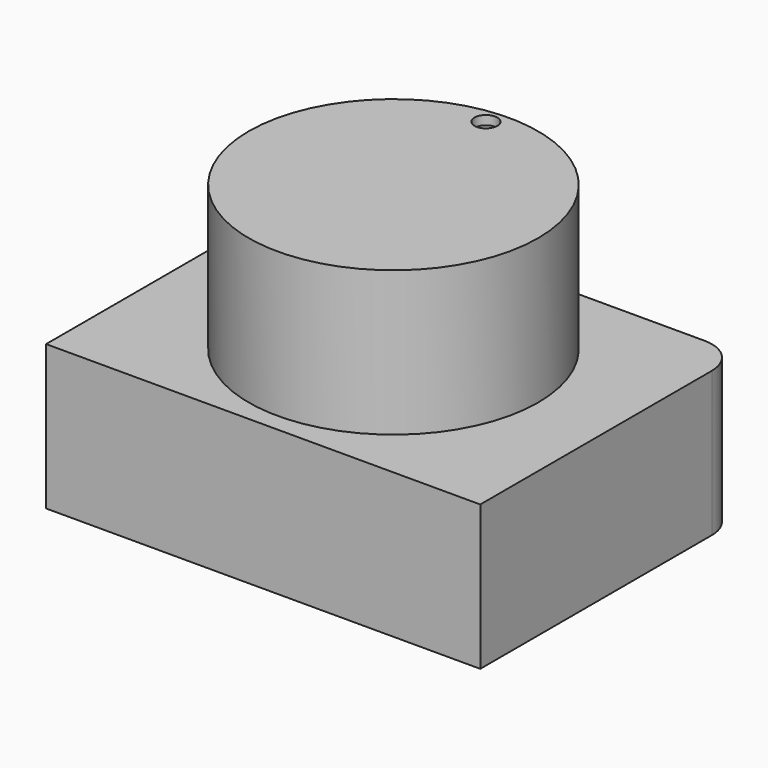
from build123d import *

# Parameters (mm, degrees)
F1_DEPTH = 25.4
F2_R     = 25.4
F3_DEPTH = 25.4
F6_DEPTH = 3.175
F7_R     = 1.9943268645
F8_DEPTH = 1.5875


# Not quite as in the source:
# - a feature of the source that left no trace in its solid (it failed there, or was rolled back) is left out


with BuildPart() as f1:
    # F0 (on Top) → F1 (new body)
    with BuildSketch(Plane.XY):
        with BuildLine():
            Line((-76.2, 0), (0, 0))
            Line((0, 0), (0, 50.8))
            ThreePointArc((0, 50.8), (-1.8598719395, 55.2901280605), (-6.35, 57.15))
            Line((-6.35, 57.15), (-69.85, 57.15))
            ThreePointArc((-69.85, 57.15), (-74.3401280605, 55.2901280605), (-76.2, 50.8))
            Line((-76.2, 50.8), (-76.2, 0))
        make_face()
    extrude(amount=F1_DEPTH)

    # F2 (on face) → F6 (cut)
    with BuildSketch(Plane.XY.offset(25.4)):
        with Locations((-38.1, 28.575)):
            Circle(F2_R)
    extrude(amount=-F6_DEPTH, mode=Mode.SUBTRACT)


with BuildPart() as f3:
    # F2 (on face) → F3 (new body)
    with BuildSketch(Plane.XY.offset(25.4)):
        with Locations((-38.1, 28.575)):
            Circle(F2_R)
    extrude(amount=F3_DEPTH)

    # F7 (on face) → F8 (cut)
    with BuildSketch(Plane.XY.offset(50.8)):
        with Locations((-39.8789197206, 51.0874353349)):
            Circle(F7_R)
    extrude(amount=-F8_DEPTH, mode=Mode.SUBTRACT)


solid = Compound([f1.part, f3.part])
